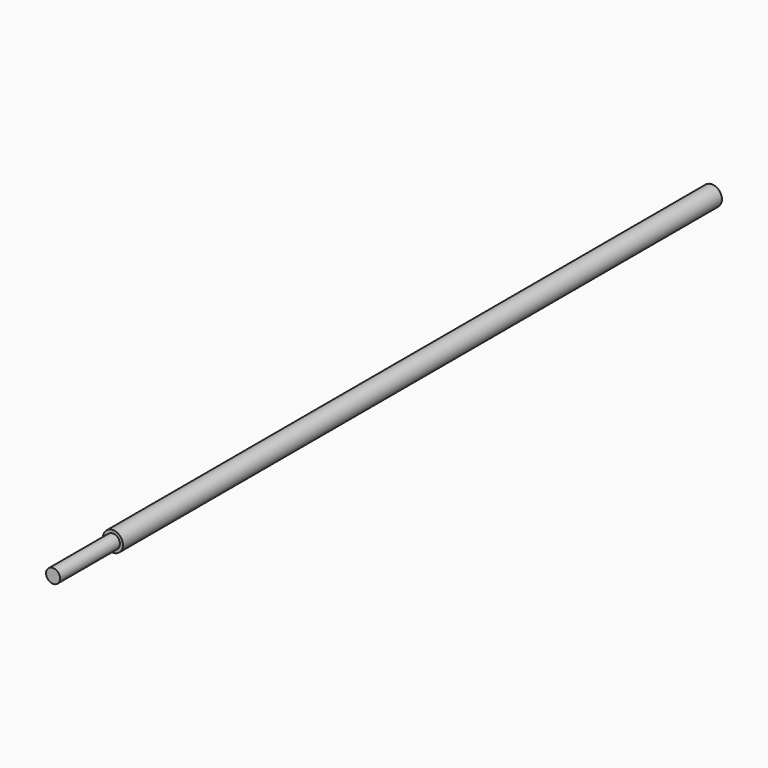
from build123d import *

# Parameters (mm, degrees)
F0_R     = 7
F1_DEPTH = 75
F2_R     = 10
F2_R_2   = 7
F3_DEPTH = 750


with BuildPart() as f1:
    # F0 (on Front) → F1 (new body)
    with BuildSketch(Plane.XZ):
        Circle(F0_R)
    extrude(amount=F1_DEPTH)

    # F2 (on face) → F3 (join)
    with BuildSketch(Plane(origin=(0, 0, 0), x_dir=(-1, 0, 0), z_dir=(0, 1, 0))):
        Circle(F2_R)
        Circle(F2_R_2, mode=Mode.SUBTRACT)
        Circle(F2_R_2)
    extrude(amount=F3_DEPTH)


solid = f1.part
